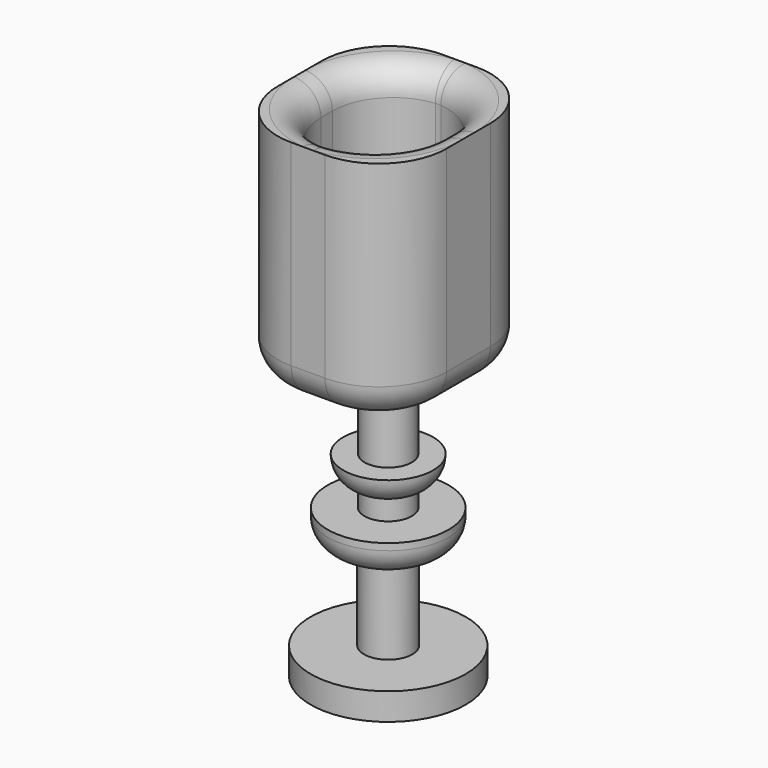
from build123d import *

# Parameters (mm, degrees)
F0_W        = 35.713232588
F0_H        = 43.3274284005
F1_DEPTH    = 31.75
F2_T        = -5.08
F3_R        = 12.7
F4_T1_DEPTH = 38.2474284005
F5_R        = 6.35
F6_R        = 5.07999
F7_R        = 4.4336766497
F8_DEPTH    = 15.24
F9_R        = 8.453024689
F10_DEPTH   = 5.08
F11_R       = 5.07999
F12_R       = 4.45495875
F13_DEPTH   = 3.81
F14_R       = 11.3706075555
F15_DEPTH   = 6.35
F16_R       = 5.08
F17_R       = 4.5498563982
F18_DEPTH   = 16.51
F19_R       = 14.5872026809
F20_DEPTH   = 5.08


# Not quite as in the source:
# - a fillet or chamfer that OpenCascade refuses, or shapes differently, is made with other operations: its cross-section is extruded or revolved along the edge and cut away or added
# - a fillet or chamfer is up to 0.001 mm smaller than in the source, because OpenCascade refuses the exact size


with BuildPart() as f1:
    # F0 (on Right) → F1 (new body)
    with BuildSketch(Plane.YZ):
        with Locations((2.1306423005, 37.6035124063)):
            Rectangle(F0_W, F0_H)
    extrude(amount=F1_DEPTH)

    # F2
    f2_openings = [f1.faces().sort_by_distance(p)[0] for p in [
        (15.875, 2.130642, 59.267227),
    ]]
    offset(amount=F2_T, openings=f2_openings)

    # F3
    f3_edges = [f1.edges().sort_by_distance(p)[0] for p in [
        (0, -15.725974, 37.603512),
        (31.75, -15.725974, 37.603512),
        (31.75, 19.987259, 37.603512),
        (0, 19.987259, 37.603512),
    ]]
    fillet(f3_edges, radius=F3_R)

    # F4: fillet of radius 11.43 on 4 edges, made by hand

    # F4_s2 → F4_t1 (join)
    with BuildSketch(Plane.XY.offset(21.0197982061)):
        with BuildLine():
            ThreePointArc((5.08, 0.7840260065), (8.427769491, -7.2982045025), (16.51, -10.6459739935))
            Line((16.51, -10.6459739935), (5.08, -10.6459739935))
            Line((5.08, -10.6459739935), (5.08, 0.7840260065))
        make_face()
        with BuildLine():
            ThreePointArc((16.51, 14.9072585945), (8.427769491, 11.5594891034), (5.08, 3.4772585945))
            Line((5.08, 3.4772585945), (5.08, 14.9072585945))
            Line((5.08, 14.9072585945), (16.51, 14.9072585945))
        make_face()
        with BuildLine():
            ThreePointArc((15.24, 14.9072585945), (23.322230509, 11.5594891034), (26.67, 3.4772585945))
            Line((26.67, 3.4772585945), (26.67, 14.9072585945))
            Line((26.67, 14.9072585945), (15.24, 14.9072585945))
        make_face()
        with BuildLine():
            ThreePointArc((15.24, -10.6459739935), (23.322230509, -7.2982045025), (26.67, 0.7840260065))
            Line((26.67, 0.7840260065), (26.67, -10.6459739935))
            Line((26.67, -10.6459739935), (15.24, -10.6459739935))
        make_face()
    extrude(amount=F4_T1_DEPTH)

    # F5
    f5_edges = [f1.edges().sort_by_distance(p)[0] for p in [
        (15.875, -15.725974, 15.939798),
        (3.719744, -12.00623, 15.939798),
        (0, 2.130642, 15.939798),
        (3.719744, 16.267515, 15.939798),
        (15.875, 19.987259, 15.939798),
        (28.030256, 16.267515, 15.939798),
        (31.75, 2.130642, 15.939798),
        (28.030256, -12.00623, 15.939798),
    ]]
    fillet(f5_edges, radius=F5_R)

    # F6 (radius 5.08 in the source; OpenCascade refuses exactly that, so slightly less here)
    f6_edges = [f1.edges().sort_by_distance(p)[0] for p in [
        (15.875, 14.889606, 40.143512),
        (26.67, 3.477259, 40.143512),
        (23.543702, 11.331775, 21.019798),
        (23.543702, 11.331775, 59.267227),
        (15.875, -10.628321, 40.143512),
        (26.67, 0.784026, 40.143512),
        (23.543702, -7.07049, 21.019798),
        (23.543702, -7.07049, 59.267227),
        (5.08, 3.477259, 40.143512),
        (8.206298, 11.331775, 21.019798),
        (8.206298, 11.331775, 59.267227),
        (5.08, 0.784026, 40.143512),
        (8.206298, -7.07049, 21.019798),
        (8.206298, -7.07049, 59.267227),
    ]]
    fillet(f6_edges, radius=F6_R)

    # F7 (on face) → F8 (join)
    with BuildSketch(Plane(origin=(0, 0, 15.9397982061), x_dir=(1, 0, 0), z_dir=(0, 0, -1))):
        with Locations((15.4130682349, -3.6905435845)):
            Circle(F7_R)
    extrude(amount=F8_DEPTH)

    # F9 (on face) → F10 (join)
    with BuildSketch(Plane(origin=(0, 0, 0.6997982061), x_dir=(1, 0, 0), z_dir=(0, 0, -1))):
        with Locations((15.4130682349, -3.6905435845)):
            Circle(F9_R)
    extrude(amount=F10_DEPTH)

    # F11 (radius 5.08 in the source; OpenCascade refuses exactly that, so slightly less here)
    f11_edges = [f1.edges().sort_by_distance(p)[0] for p in [
        (6.960044, 3.690544, -4.380202),
    ]]
    fillet(f11_edges, radius=F11_R)

    # F12 (on face) → F13 (join)
    with BuildSketch(Plane(origin=(0, 0, -4.3802017939), x_dir=(1, 0, 0), z_dir=(0, 0, -1))):
        with Locations((15.4130682349, -3.6905435845)):
            Circle(F12_R)
    extrude(amount=F13_DEPTH)

    # F14 (on face) → F15 (join)
    with BuildSketch(Plane(origin=(0, 0, -8.1902017939), x_dir=(1, 0, 0), z_dir=(0, 0, -1))):
        with Locations((15.4130682349, -3.6905435845)):
            Circle(F14_R)
    extrude(amount=F15_DEPTH)

    # F16
    f16_edges = [f1.edges().sort_by_distance(p)[0] for p in [
        (4.042461, 3.690544, -14.540202),
    ]]
    fillet(f16_edges, radius=F16_R)

    # F17 (on face) → F18 (join)
    with BuildSketch(Plane(origin=(0, 0, -14.5402017939), x_dir=(1, 0, 0), z_dir=(0, 0, -1))):
        with Locations((15.4130682349, -3.6905435845)):
            Circle(F17_R)
    extrude(amount=F18_DEPTH)

    # F19 (on face) → F20 (join)
    with BuildSketch(Plane(origin=(0, 0, -31.0502017939), x_dir=(1, 0, 0), z_dir=(0, 0, -1))):
        with Locations((15.4130682349, -3.6905435845)):
            Circle(F19_R)
    extrude(amount=F20_DEPTH)


solid = f1.part
